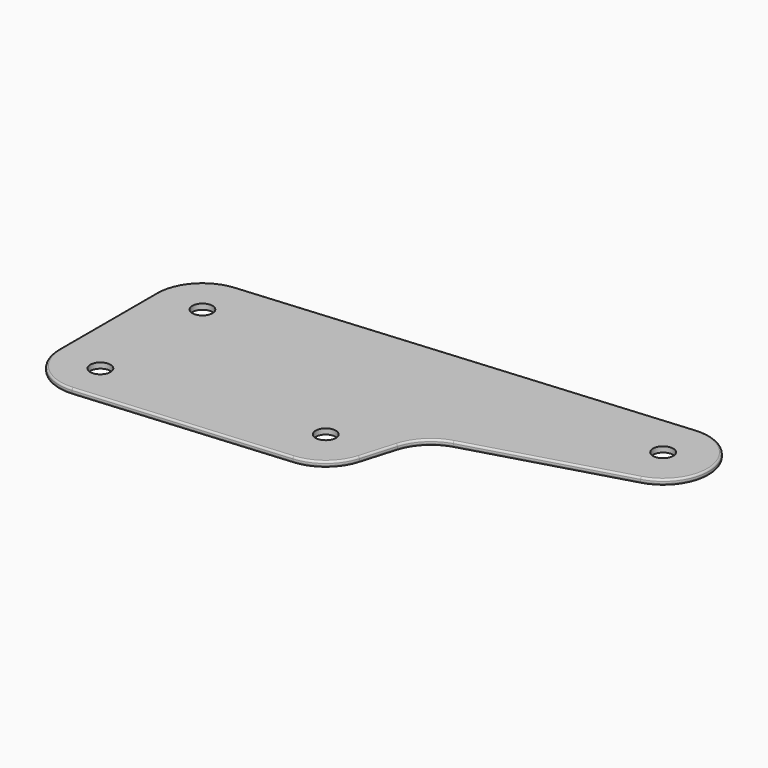
from build123d import *

# Parameters (mm, degrees)
F0_R     = 5.5
F1_DEPTH = 3
F2_R     = 1


# Not quite as in the source:
# - a feature names something its author has since deleted; it is built from what else it names


with BuildPart() as f1:
    # F0 (on Top) → F1 (new body)
    with BuildSketch(Plane.XY):
        with BuildLine():
            ThreePointArc((-114.9011806829, 81.9265817605), (-131.2129171427, 73.936702076), (-137.8111356168, 57.0141007194))
            Line((-137.8111356168, 57.0141007194), (-137.8111356168, -9.4738897749))
            ThreePointArc((-137.8111356168, -9.4738897749), (-129.7329640684, -27.8763820478), (-110.7189978684, -34.3861951608))
            Line((-110.7189978684, -34.3861951608), (2.0921377484, -24.9123053859))
            ThreePointArc((2.0921377484, -24.9123053859), (15.7854299835, -19.3860826429), (23.9716178382, -7.0965863779))
            Line((23.9716178382, -7.0965863779), (29.5724079217, 11.8223687823))
            ThreePointArc((29.5724079217, 11.8223687823), (35.9169319793, 22.4538833983), (46.5845244365, 28.7375574602))
            Line((46.5845244365, 28.7375574602), (129.3918966116, 52.7381994328))
            ThreePointArc((129.3918966116, 52.7381994328), (147.0153896078, 81.2971043835), (120.3423502221, 101.6624555296))
            Line((120.3423502221, 101.6624555296), (-114.9011806829, 81.9265817605))
        make_face()
        with Locations((-112.8111356168, -12.4858992806)):
            Circle(F0_R, mode=Mode.SUBTRACT)
        Circle(F0_R, mode=Mode.SUBTRACT)
        with Locations((-112.8111356168, 57.0141007194)):
            Circle(F0_R, mode=Mode.SUBTRACT)
        with Locations((122.4323952882, 76.7499744885)):
            Circle(F0_R, mode=Mode.SUBTRACT)
    extrude(amount=F1_DEPTH)

    # F2
    f2_edges = [f1.edges().sort_by_distance(p)[0] for p in [
        (2.720585, 91.794519, 0),
        (147.01539, 81.297104, 0),
        (87.988211, 40.737878, 0),
        (-137.811136, 23.770105, 0),
        (-137.811136, 23.770105, 3),
        (-131.212917, 73.936702, 0),
        (-131.212917, 73.936702, 3),
        (2.720585, 91.794519, 3),
        (147.01539, 81.297104, 3),
        (87.988211, 40.737878, 3),
    ]]
    fillet(f2_edges, radius=F2_R)


solid = f1.part
